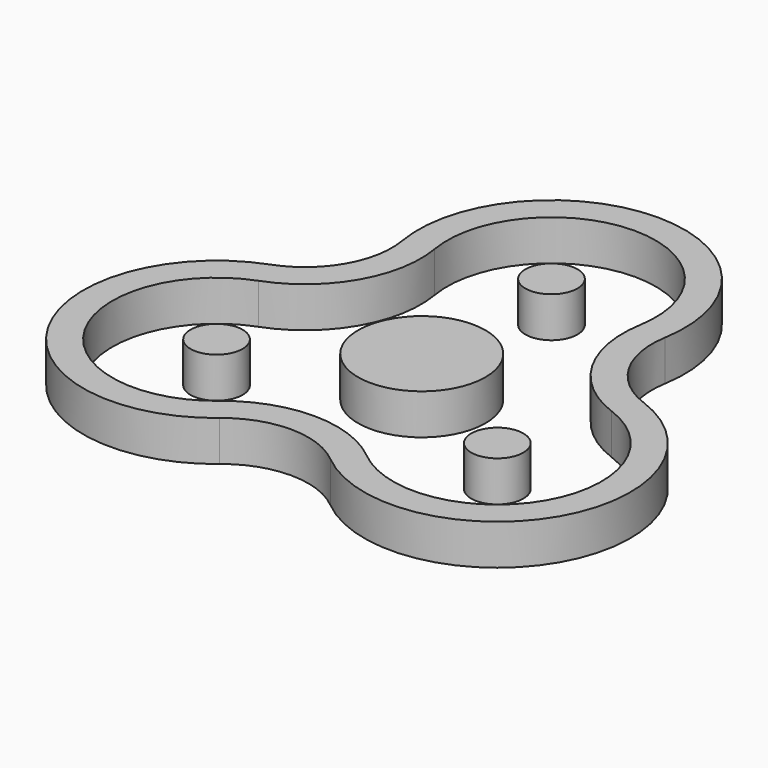
from build123d import *

# Parameters (mm, degrees)
F1_DEPTH = 7
F0_R     = 11
F0_R_2   = 4.5


# Not quite as in the source:
# - ends of sketch curves that miss each other by under 0.0002 mm in the source are joined


with BuildPart() as f1:
    # F0 (on Top) → F1 (new body)
    with BuildSketch(Plane.XY):
        with BuildLine():
            ThreePointArc((32.2462730801, 7.5647624351), (24.4716930106, 14.1287385472), (22.6744129825, 24.1437104471))
            ThreePointArc((22.6744129825, 24.1437104471), (0, 51), (-22.6744135565, 24.1437103495))
            ThreePointArc((-22.6744135565, 24.1437103495), (-24.4716930106, 14.1287385472), (-32.2462730801, 7.5647624351))
            ThreePointArc((-32.2462730801, 7.5647624351), (-44.167295593, -25.5), (-9.571859726, -31.7084733306))
            ThreePointArc((-9.571859726, -31.7084733306), (0, -28.2574780285), (9.5718595015, -31.7084736015))
            ThreePointArc((9.5718595015, -31.7084736015), (44.167295593, -25.5), (32.2462730801, 7.5647624351))
        make_face()
        with BuildLine():
            ThreePointArc((-12.7624796347, -27.8588052153), (-39.8371685741, -23), (-30.5076728529, 2.8767710287))
            ThreePointArc((-30.5076728529, 2.8767710287), (-20.1415664959, 11.6287388383), (-17.7451932181, 24.9820341866))
            ThreePointArc((-17.7451932181, 24.9820341866), (0, 46), (17.7451932181, 24.9820341866))
            ThreePointArc((17.7451932181, 24.9820341866), (20.1415664959, 11.6287388383), (30.5076728529, 2.8767710287))
            ThreePointArc((30.5076728529, 2.8767710287), (39.8371685741, -23), (12.7624796347, -27.8588052153))
            ThreePointArc((12.7624796347, -27.8588052153), (0, -23.2574776767), (-12.7624796347, -27.8588052153))
        make_face(mode=Mode.SUBTRACT)
    extrude(amount=F1_DEPTH)


with BuildPart() as f1b:
    # F0 (on Top) → F1, piece 2 (new body)
    with BuildSketch(Plane.XY):
        Circle(F0_R)
    extrude(amount=F1_DEPTH)


with BuildPart() as f1c:
    # F0 (on Top) → F1, piece 3 (new body)
    with BuildSketch(Plane.XY):
        with Locations((-24.248711306, -14)):
            Circle(F0_R_2)
    extrude(amount=F1_DEPTH)


with BuildPart() as f1d:
    # F0 (on Top) → F1, piece 4 (new body)
    with BuildSketch(Plane.XY):
        with Locations((24.248711306, -14)):
            Circle(F0_R_2)
    extrude(amount=F1_DEPTH)


with BuildPart() as f1e:
    # F0 (on Top) → F1, piece 5 (new body)
    with BuildSketch(Plane.XY):
        with Locations((0, 28)):
            Circle(F0_R_2)
    extrude(amount=F1_DEPTH)


solid = Compound([f1.part, f1b.part, f1c.part, f1d.part, f1e.part])
